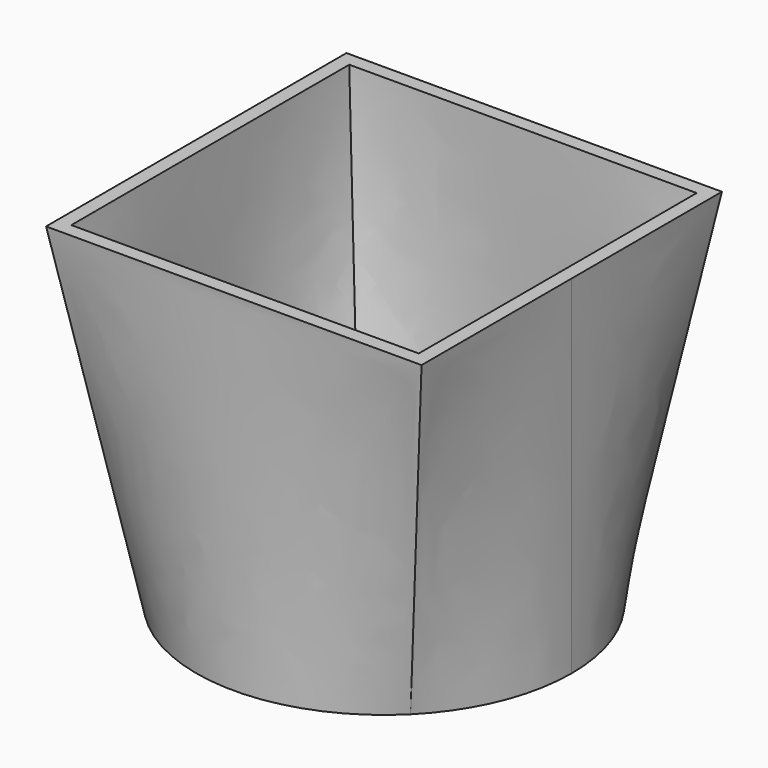
from build123d import *

# Parameters (mm, degrees)
F0_R = 27
F2_W = 54
F2_H = 54
F4_T = 2


# Not quite as in the source:
# - a shell that OpenCascade refuses in one call is made with other operations: the cavity is built on its own and cut out


with BuildPart() as f3:
    # F0 (on Top) → F3 section 0
    with BuildSketch(Plane.XY):
        Circle(F0_R)
    # F2 (on offset) → F3 section 1
    with BuildSketch(Plane.XY.offset(50)):
        Rectangle(F2_W, F2_H)
    loft()

    # F4: shell of thickness 2, made by hand


with BuildPart() as f4_core1:
    # F4_t2: copy of F3
    add(f3.part)

    # the walls: a layer under each face that stays
    f4_faces = [f4_core1.faces().sort_by_distance(p)[0] for p in [
        (25.9723736862, 11.9162263358, 25),
        (0, 26.999999999, 25),
        (-26.999999999, 0, 25),
        (0, -26.999999999, 25),
        (25.9723736862, -11.9162263358, 25),
        (0, 0, 0),
    ]]
    thicken(f4_faces, amount=-F4_T, mode=Mode.SUBTRACT)


with BuildPart() as f3_1:
    add(f3.part)

    # what is left inside the walls is the cavity
    f4_cavity = [f4_core1.part.solids().sort_by_distance(p)[0] for p in [
        (4.996272, 9.992544, 49.98),
    ]]
    add(f4_cavity, mode=Mode.SUBTRACT)


solid = f3_1.part
